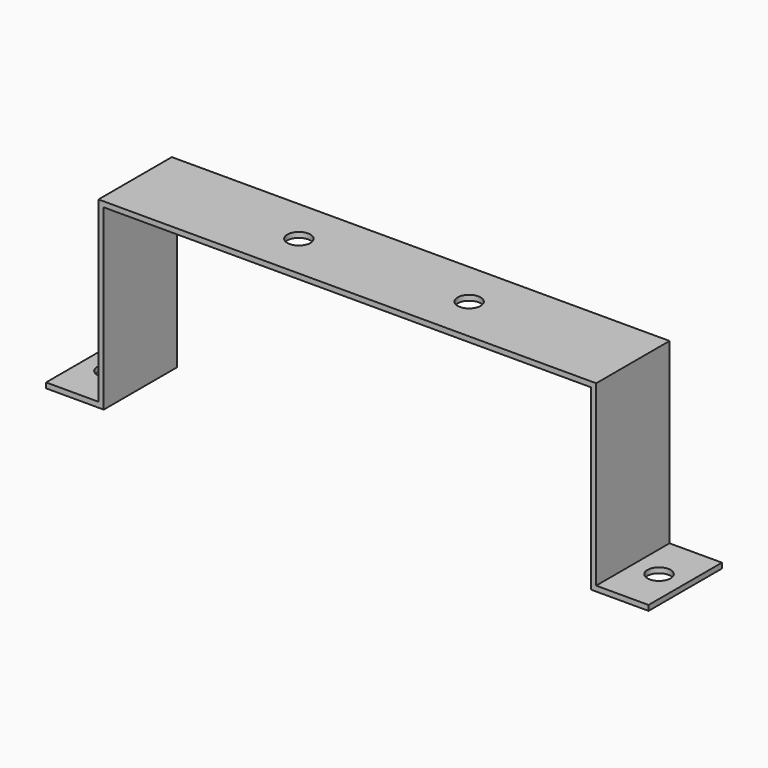
from build123d import *

# Parameters (mm, degrees)
F1_DEPTH = 17.5
F2_R     = 4.4
F3_DEPTH = 25
F4_R     = 4.4
F5_DEPTH = 25


# Not quite as in the source:
# - a feature names something its author has since deleted; it is built from what else it names


with BuildPart() as f1:
    # F0 (on Front) → F1 (new body, symmetric)
    with BuildSketch(Plane.XZ):
        Polygon((95, -38), (95, 30), (-95, 30), (-95, -38), (-115, -38), (-115, -40), (-93, -40), (-93, 28), (93, 28), (93, -40), (115, -40), (115, -38), align=None)
    extrude(amount=F1_DEPTH, both=True)

    # F2 (on face) → F3 (cut)
    with BuildSketch(Plane.XY.offset(-38)):
        with Locations((-105, 0)):
            Circle(F2_R)
        with Locations((105, 0)):
            Circle(F2_R)
    extrude(amount=-F3_DEPTH, mode=Mode.SUBTRACT)

    # F4 (on face) → F5 (cut)
    with BuildSketch(Plane.XY.offset(30)):
        with Locations((-32.5, 0)):
            Circle(F4_R)
        with Locations((32.5, 0)):
            Circle(F4_R)
    extrude(amount=-F5_DEPTH, mode=Mode.SUBTRACT)


solid = f1.part
